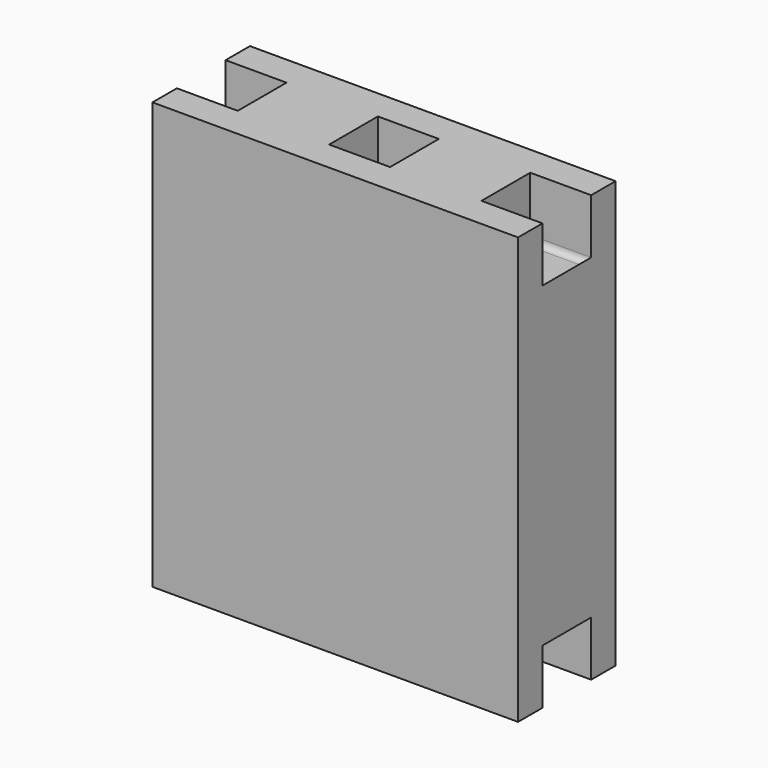
from build123d import *

# Parameters (mm, degrees)
F0_W      = 76.2
F0_H      = 88.9
F1_DEPTH  = 12.7
F4_DEPTH  = 12.7
F2_W      = 12.7
F2_H      = 12.7
F3_W      = 12.7
F3_H      = 12.7
F5_DEPTH  = 12.7
F6_R      = 1.27
F7_DEPTH  = 12.7
F8_R      = 7.9375
F9_DEPTH  = 12.7
F10_R     = 9.525
F11_DEPTH = 6.35
F12_SIZE2 = 1.26999
F12_SIZE  = 3.17499


# Not quite as in the source:
# - a fillet or chamfer is up to 0.001 mm smaller than in the source, because OpenCascade refuses the exact size


with BuildPart() as f1:
    # F0 (on Front) → F1 (new body, symmetric)
    with BuildSketch(Plane.XZ):
        Rectangle(F0_W, F0_H)
    extrude(amount=F1_DEPTH, both=True)

    # F4 (add, symmetric): faces of the model
    f4_faces = [f1.faces().sort_by_distance(p)[0] for p in [
        (-38.1, 0, 0),
        (38.1, 0, 0),
    ]]
    extrude(f4_faces, amount=F4_DEPTH, both=True, dir=(-1, 0, 0))

    # F2 (on face) + F3 (on face) → F5 (cut, symmetric)
    with BuildSketch(Plane.XY.offset(44.45)):
        with Locations((-31.75, 0)):
            Rectangle(F2_W, F2_H)
        Rectangle(F2_W, F2_H)
        with Locations((31.75, 0)):
            Rectangle(F2_W, F2_H)
    with BuildSketch(Plane(origin=(0, 0, -44.45), x_dir=(1, 0, 0), z_dir=(0, 0, -1))):
        with Locations((-31.75, 0)):
            Rectangle(F3_W, F3_H)
        Rectangle(F3_W, F3_H)
        with Locations((31.75, 0)):
            Rectangle(F3_W, F3_H)
    extrude(amount=F5_DEPTH, both=True, dir=(0, 0, 1), mode=Mode.SUBTRACT)

    # F6
    f6_edges = [f1.edges().sort_by_distance(p)[0] for p in [
        (-38.1, 0, 31.75),
        (-31.75, -6.35, 31.75),
        (-25.4, 0, 31.75),
        (-31.75, 6.35, 31.75),
        (-6.35, 0, 31.75),
        (0, -6.35, 31.75),
        (6.35, 0, 31.75),
        (0, 6.35, 31.75),
        (31.75, -6.35, 31.75),
        (38.1, 0, 31.75),
        (31.75, 6.35, 31.75),
        (25.4, 0, 31.75),
        (-31.75, 6.35, -31.75),
        (-25.4, 0, -31.75),
        (-31.75, -6.35, -31.75),
        (-38.1, 0, -31.75),
        (6.35, 0, -31.75),
        (0, -6.35, -31.75),
        (-6.35, 0, -31.75),
        (0, 6.35, -31.75),
        (31.75, 6.35, -31.75),
        (38.1, 0, -31.75),
        (31.75, -6.35, -31.75),
        (25.4, 0, -31.75),
    ]]
    fillet(f6_edges, radius=F6_R)

    # F7 (cut, symmetric): faces of the model
    f7_faces = [f1.faces().sort_by_distance(p)[0] for p in [
        (50.8, 0, 0),
        (-50.8, 0, 0),
    ]]
    extrude(f7_faces, amount=F7_DEPTH, both=True, dir=(1, 0, 0), mode=Mode.SUBTRACT)

    # F8 (on face) → F9 (cut)
    with BuildSketch(Plane(origin=(0, 12.7, 0), x_dir=(-1, 0, 0), z_dir=(0, 1, 0))):
        Circle(F8_R)
    extrude(amount=-F9_DEPTH, mode=Mode.SUBTRACT)

    # F10 (on face) → F11 (cut)
    with BuildSketch(Plane(origin=(0, 0, 0), x_dir=(-1, 0, 0), z_dir=(0, 1, 0))):
        Circle(F10_R)
    extrude(amount=F11_DEPTH, mode=Mode.SUBTRACT)

    # F12 (size 3.175 and 1.27 in the source; OpenCascade refuses exactly that, so slightly less here)
    f12_edges = [f1.edges().sort_by_distance(p)[0] for p in [
        (9.525, 0, 0),
        (9.525, 6.35, 0),
    ]]
    f12_side = f1.faces().sort_by_distance((9.525, 3.175, 0))[0]
    chamfer(f12_edges, length=F12_SIZE, length2=F12_SIZE2, reference=f12_side)


solid = f1.part
